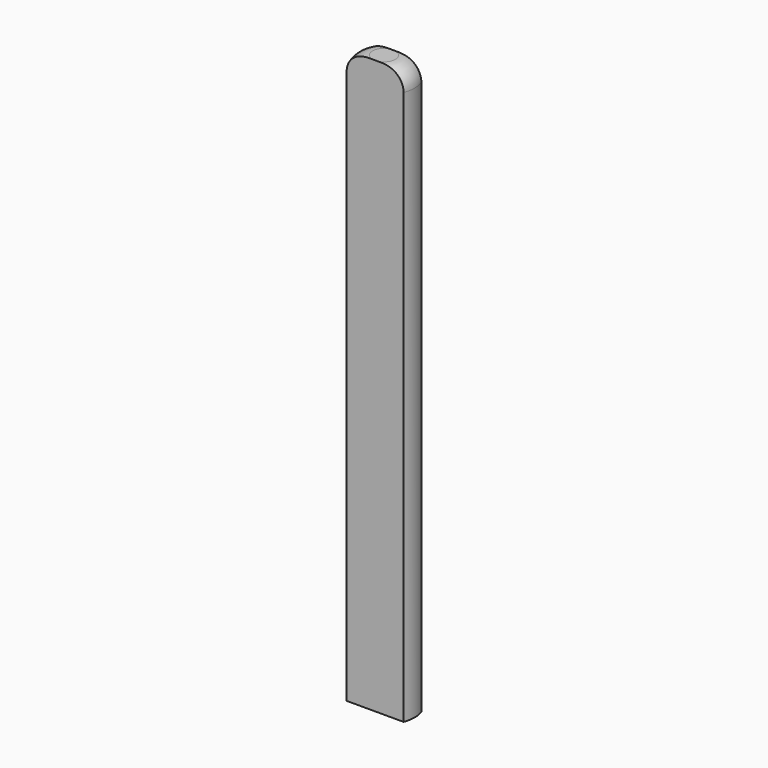
from build123d import *

# Parameters (mm, degrees)
F1_DEPTH = 150
F2_R     = 5
F3_R     = 5


# Not quite as in the source:
# - a feature names something its author has since deleted; it is built from what else it names


with BuildPart() as f1:
    # F0 (on Top) → F1 (new body)
    with BuildSketch(Plane.XY):
        with BuildLine():
            Line((7.4523278298, 2.9090909091), (-7.4523278298, 2.9090909091))
            ThreePointArc((-7.4523278298, 2.9090909091), (-8, 0), (-7.4523278298, -2.9090909091))
            Line((-7.4523278298, -2.9090909091), (7.4523278298, -2.9090909091))
            ThreePointArc((7.4523278298, -2.9090909091), (8, 0), (7.4523278298, 2.9090909091))
        make_face()
    extrude(amount=F1_DEPTH)

    # F2
    f2_edges = [f1.edges().sort_by_distance(p)[0] for p in [
        (8, 0, 150),
    ]]
    fillet(f2_edges, radius=F2_R)

    # F3
    f3_edges = [f1.edges().sort_by_distance(p)[0] for p in [
        (-8, 0, 150),
    ]]
    fillet(f3_edges, radius=F3_R)


solid = f1.part
